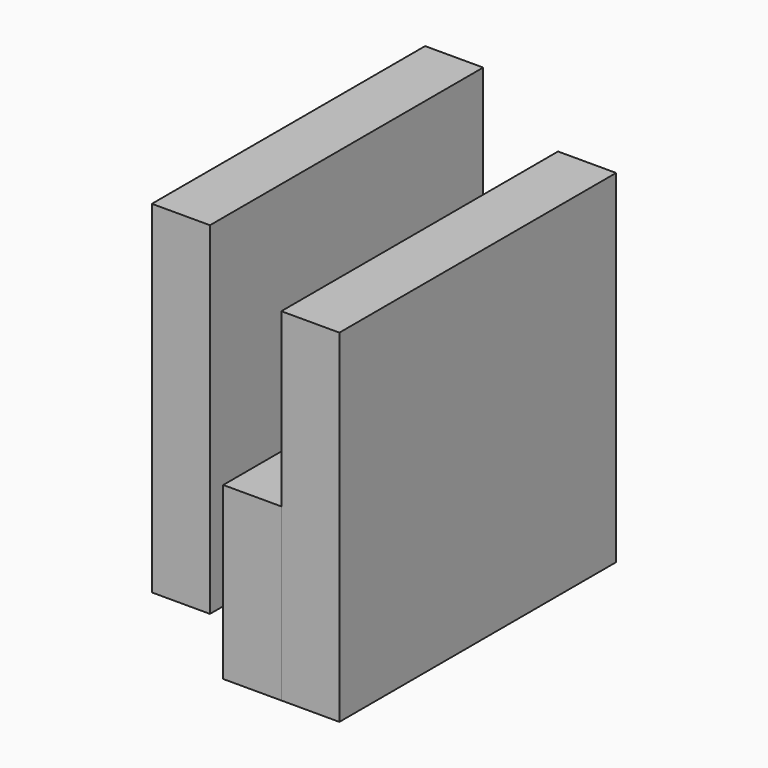
from build123d import *

# Parameters (mm, degrees)
F0_W     = 75.5894184113
F0_H     = 75.1656368375
F0_W_2   = 75.6931006908
F1_DEPTH = 25.4
F2_W     = 58.5926715285
F2_H     = 41.5871664882
F2_W_2   = 8.5760951042
F2_H_2   = 8.3214826882
F2_W_3   = 8.4206517786
F3_DEPTH = 25.4
F4_W     = 91.1564920098
F4_H     = 141.0772651434
F4_H_2   = 8.5697695613
F5_DEPTH = 25.4


with BuildPart() as f1:
    # F0 (on Right) → F1 (new body)
    with BuildSketch(Plane.YZ):
        with Locations((-37.7947092056, 37.5828184187)):
            Rectangle(F0_W, F0_H)
        with Locations((37.8465503454, 37.5828184187)):
            Rectangle(F0_W_2, F0_H)
        Polygon((0, 0), (-75.5894184113, 0), (-75.5894184113, -74.7117847204), (75.6931006908, -74.7117847204), (75.6931006908, 0), align=None)
    extrude(amount=F1_DEPTH)

    # F2 (on face) → F3 (join)
    with BuildSketch(Plane(origin=(0, 0, 0), x_dir=(0, -1, 0), z_dir=(-1, 0, 0))):
        with Locations((46.293082647, -53.9182014763)):
            Rectangle(F2_W, F2_H)
        Polygon((0, -74.7117847204), (16.9967468828, -74.7117847204), (16.9967468828, -33.1246182323), (16.9967468828, -22.4458947778), (0, -22.4458947778), align=None)
        Polygon((16.9967468828, -33.1246182323), (75.5894184113, -33.1246182323), (75.5894184113, -20.1201699674), (16.9967468828, -20.1201699674), (16.9967468828, -22.4458947778), align=None)
        Polygon((16.9967468828, -20.1201699674), (75.5894184113, -20.1201699674), (75.5894184113, 0), (16.9967468828, 0), (16.9967468828, -8.3214826882), align=None)
        Polygon((0, -22.4458947778), (16.9967468828, -22.4458947778), (16.9967468828, -20.1201699674), (8.5760951042, -20.1201699674), (8.5760951042, -8.3214826882), (0, -8.3214826882), align=None)
        with Locations((4.2880475521, -4.1607413441)):
            Rectangle(F2_W_2, F2_H_2)
        with Locations((12.7864209935, -4.1607413441)):
            Rectangle(F2_W_3, F2_H_2)
    extrude(amount=F3_DEPTH)

    # F4 (on face) → F5 (join)
    with BuildSketch(Plane(origin=(-25.4, 0, 0), x_dir=(0, -1, 0), z_dir=(-1, 0, 0))):
        with Locations((-20.9354860708, 23.8422006369)):
            Rectangle(F4_W, F4_H)
        Polygon((24.6427599341, 102.9506027699), (24.6427599341, 94.3808332086), (24.6427599341, -46.6964319348), (82.840628922, -46.6964319348), (82.840628922, 102.9506027699), align=None)
        with Locations((-20.9354860708, 98.6657179892)):
            Rectangle(F4_W, F4_H_2)
    extrude(amount=F5_DEPTH)


solid = f1.part
